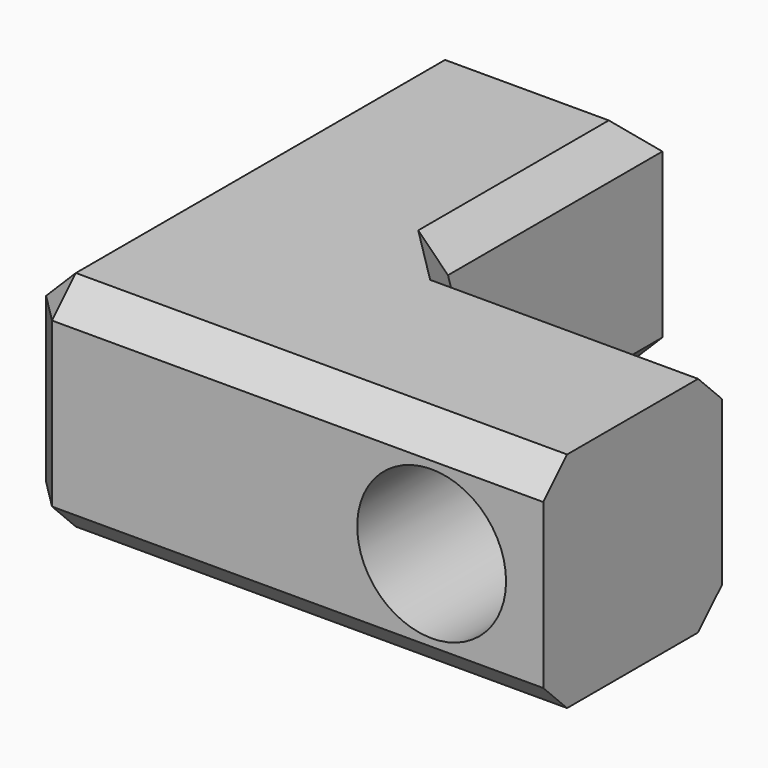
from build123d import *

# Parameters (mm, degrees)
F1_DEPTH = 19.05
F2_SIZE  = 2.54
F4_D     = 12.7


with BuildPart() as f1:
    # F0 (on Top) → F1 (new body)
    with BuildSketch(Plane.XY):
        Polygon((-19.2860513926, 35.6976958707), (-38.3360513926, 35.6976958707), (-38.3360513926, -8.7523041293), (6.1139486074, -8.7523041293), (6.1139486074, 10.2976958707), (-19.2860513926, 10.2976958707), align=None)
    extrude(amount=F1_DEPTH)

    # F2
    f2_edges = [f1.edges().sort_by_distance(p)[0] for p in [
        (-19.286051, 10.297696, 9.525),
        (-28.811051, 35.697696, 19.05),
        (-38.336051, 13.472696, 19.05),
        (-16.111051, -8.752304, 19.05),
        (-38.336051, 13.472696, 0),
        (-38.336051, -8.752304, 9.525),
        (-16.111051, -8.752304, 0),
        (-6.586051, 10.297696, 0),
        (-6.586051, 10.297696, 19.05),
        (-19.286051, 22.997696, 0),
        (-19.286051, 22.997696, 19.05),
    ]]
    chamfer(f2_edges, length=F2_SIZE)

    # F4 (through all)
    with Locations(Plane(origin=(0, 10.2976958707, 0), x_dir=(-1, 0, 0), z_dir=(0, 1, 0))):
        with Locations((3.4110513926, 9.525)):
            Hole(F4_D / 2)


solid = f1.part
